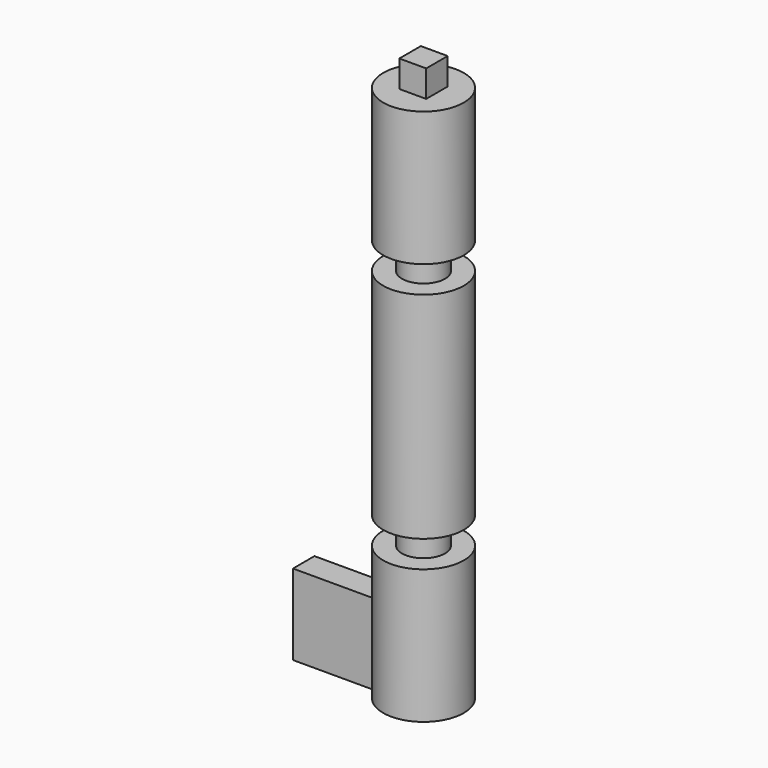
from build123d import *

# Parameters (mm, degrees)
F0_R      = 7.5
F1_DEPTH  = 20
F2_R      = 4
F3_DEPTH  = 5
F4_R      = 7.5
F4_R_2    = 4
F5_DEPTH  = 25
F7_W      = 5
F7_H      = 5
F8_DEPTH  = 5
F9_W      = 24.7944914738
F9_H      = 5
F10_DEPTH = 15


with BuildPart() as f1:
    # F0 (on Top) → F1 (new body)
    with BuildSketch(Plane.XY):
        Circle(F0_R)
    extrude(amount=F1_DEPTH)

    # F2 (on face) → F3 (join)
    with BuildSketch(Plane.XY.offset(20)):
        Circle(F2_R)
    extrude(amount=F3_DEPTH)

    # F4 (on face) → F5 (join)
    with BuildSketch(Plane.XY.offset(25)):
        Circle(F4_R)
        Circle(F4_R_2, mode=Mode.SUBTRACT)
        Circle(F4_R_2)
    extrude(amount=F5_DEPTH)

    # F6: F1 across plane


with BuildPart() as f1_1:
    add(f1.part)
    add(f1.part.mirror(Plane.XY))

    # F7 (on face) → F8 (join)
    with BuildSketch(Plane.XY.offset(50)):
        Rectangle(F7_W, F7_H)
    extrude(amount=F8_DEPTH)

    # F9 (on face) → F10 (join)
    with BuildSketch(Plane(origin=(0, 0, -50), x_dir=(1, 0, 0), z_dir=(0, 0, -1))):
        with Locations((-9.8972457369, 0)):
            Rectangle(F9_W, F9_H)
    extrude(amount=-F10_DEPTH)


solid = f1_1.part
